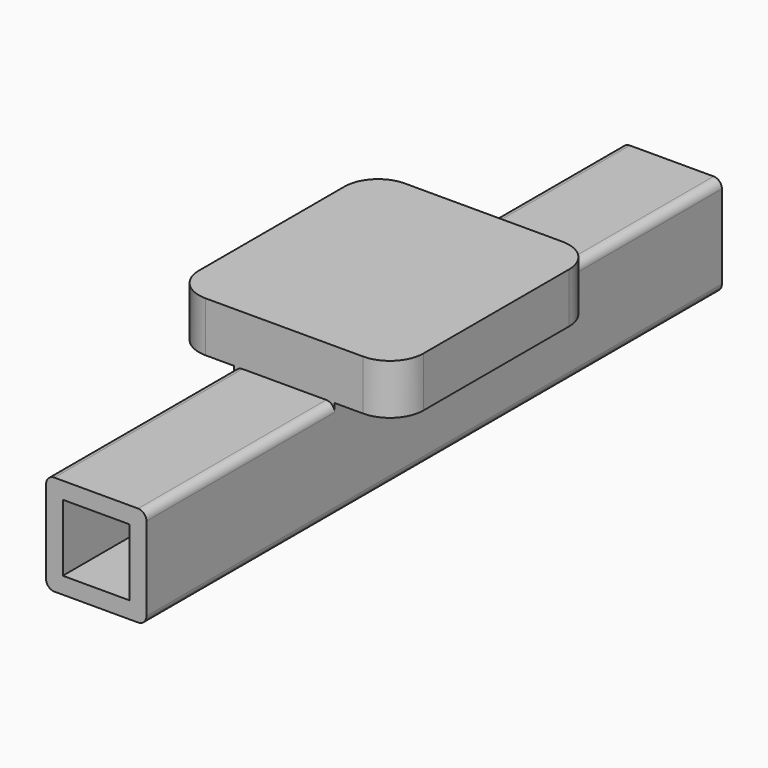
from build123d import *

# Parameters (mm, degrees)
F0_W     = 19.05
F0_H     = 19.05
F0_W_2   = 12.7
F0_H_2   = 12.7
F1_DEPTH = 136.525
F2_W     = 42.5958
F2_H     = 47.244
F3_DEPTH = 9.525
F4_R     = 6.35
F5_R     = 1.5875


with BuildPart() as f1:
    # F0 (on Front) → F1 (new body)
    with BuildSketch(Plane.XZ):
        with Locations((68.0290833116, -52.153282702)):
            Rectangle(F0_W, F0_H)
        with Locations((68.0290833116, -52.153282702)):
            Rectangle(F0_W_2, F0_H_2, mode=Mode.SUBTRACT)
    extrude(amount=-F1_DEPTH)

    # F2 (on face) → F3 (join)
    with BuildSketch(Plane.XY.offset(-42.628282702)):
        with Locations((68.0290833116, 68.2625)):
            Rectangle(F2_W, F2_H)
    extrude(amount=F3_DEPTH)

    # F4
    f4_edges = [f1.edges().sort_by_distance(p)[0] for p in [
        (89.326983, 44.6405, -37.865783),
        (89.326983, 91.8845, -37.865783),
        (46.731183, 44.6405, -37.865783),
        (46.731183, 91.8845, -37.865783),
    ]]
    fillet(f4_edges, radius=F4_R)

    # F5
    f5_edges = [f1.edges().sort_by_distance(p)[0] for p in [
        (77.554083, 68.2625, -61.678283),
        (58.504083, 68.2625, -61.678283),
        (58.504083, 22.32025, -42.628283),
        (77.554083, 22.32025, -42.628283),
        (58.504083, 114.20475, -42.628283),
        (77.554083, 114.20475, -42.628283),
    ]]
    fillet(f5_edges, radius=F5_R)


solid = f1.part
